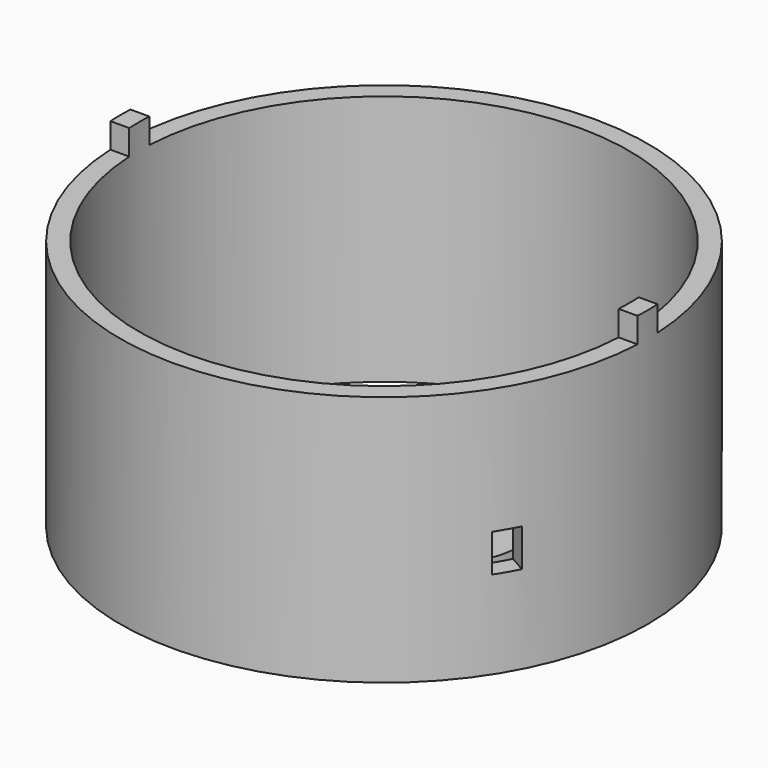
from build123d import *

# Parameters (mm, degrees)
F0_R      = 21
F0_R_2    = 19.5
F1_DEPTH  = 20
F2_W      = 2
F2_H      = 2
F3_DEPTH  = 25
F4_R      = 19.5
F5_DEPTH  = 25
F6_R      = 25.0510774743
F6_R_2    = 21
F7_DEPTH  = 2.001
F8_R      = 12
F8_R_2    = 8.5
F9_DEPTH  = 3
F16_W     = 2
F16_H     = 3
F17_DEPTH = 21.001
F18_W     = 2
F18_H     = 3
F19_DEPTH = 28.6875334795
F20_W     = 2
F20_H     = 3
F21_DEPTH = 28.6875334795


# Not quite as in the source:
# - a feature of the source that left no trace in its solid (it failed there, or was rolled back) is left out


with BuildPart() as f1:
    # F0 (on Top) → F1 (new body)
    with BuildSketch(Plane.XY):
        Circle(F0_R)
        Circle(F0_R_2, mode=Mode.SUBTRACT)
    extrude(amount=F1_DEPTH)

    # F2 (on Right) → F3 (join, symmetric)
    with BuildSketch(Plane.YZ):
        with Locations((0, 21)):
            Rectangle(F2_W, F2_H)
    extrude(amount=F3_DEPTH, both=True)

    # F4 (on face) → F5 (cut)
    with BuildSketch(Plane.XY.offset(22)):
        Circle(F4_R)
    extrude(amount=-F5_DEPTH, mode=Mode.SUBTRACT)

    # F6 (on face) → F7 (cut, through all)
    with BuildSketch(Plane.XY.offset(20)):
        Circle(F6_R)
        Circle(F6_R_2, mode=Mode.SUBTRACT)
    extrude(amount=F7_DEPTH, mode=Mode.SUBTRACT)

    # F16 (on Front) → F17 (cut, through all)
    with BuildSketch(Plane.XZ):
        with Locations((-21, 8.5)):
            Rectangle(F16_W, F16_H)
    extrude(amount=-F17_DEPTH, mode=Mode.SUBTRACT)

    # F18 (on face) → F19 (cut, through all)
    with BuildSketch(Plane(origin=(0, 0, 0), x_dir=(0.5, 0.8660254038, 0), z_dir=(0.8660254038, -0.5, 0))):
        with Locations((0, 8.5)):
            Rectangle(F18_W, F18_H)
    extrude(amount=F19_DEPTH, mode=Mode.SUBTRACT)

    # F20 (on face) → F21 (cut, through all)
    with BuildSketch(Plane(origin=(0, 0, 0), x_dir=(-0.5, 0.8660254038, 0), z_dir=(0.8660254038, 0.5, 0))):
        with Locations((0, 8.5)):
            Rectangle(F20_W, F20_H)
    extrude(amount=-F21_DEPTH, mode=Mode.SUBTRACT)


with BuildPart() as f9:
    # F8 (on face) → F9 (new body)
    with BuildSketch(Plane(origin=(0, 0, 0), x_dir=(1, 0, 0), z_dir=(0, 0, -1))):
        Circle(F8_R)
        Circle(F8_R_2, mode=Mode.SUBTRACT)
    extrude(amount=-F9_DEPTH)


solid = Compound([f1.part, f9.part])
